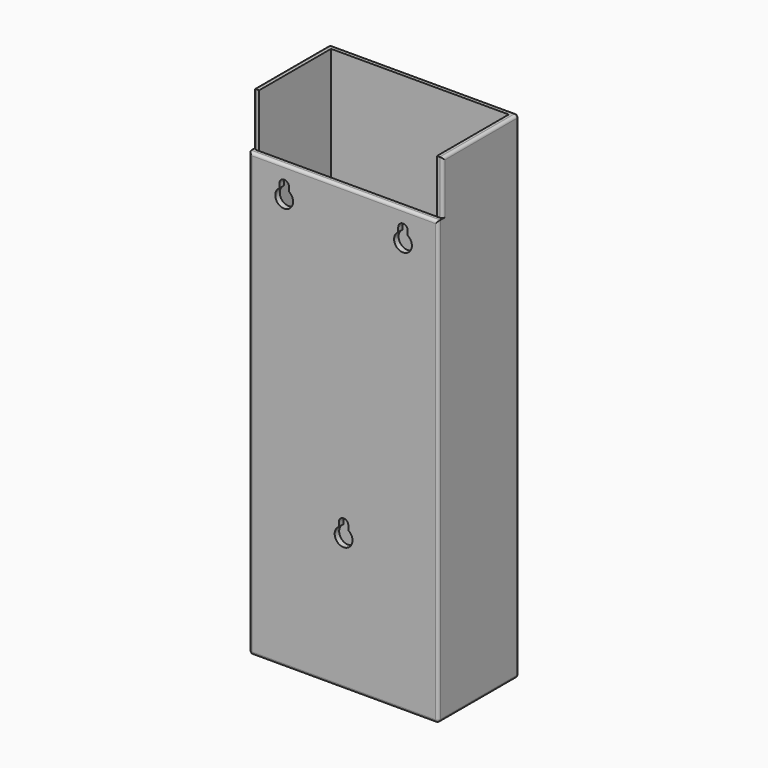
from build123d import *

# Parameters (mm, degrees)
F0_W     = 101
F0_H     = 54
F1_DEPTH = 132.5
F2_T     = -3
F3_W     = 101
F3_H     = 28.575
F4_DEPTH = 3
F6_DEPTH = 3
F7_R     = 1.5


with BuildPart() as f1:
    # F0 (on Top) → F1 (new body, symmetric)
    with BuildSketch(Plane.XY):
        Rectangle(F0_W, F0_H)
    extrude(amount=F1_DEPTH, both=True)

    # F2
    f2_openings = [f1.faces().sort_by_distance(p)[0] for p in [
        (0, 0, 132.5),
    ]]
    offset(amount=F2_T, openings=f2_openings)

    # F3 (on face) → F4 (cut, through all)
    with BuildSketch(Plane.XZ.offset(27)):
        with Locations((0, 118.2125)):
            Rectangle(F3_W, F3_H)
    extrude(amount=-F4_DEPTH, mode=Mode.SUBTRACT)

    # F5 (on face) → F6 (cut, through all)
    with BuildSketch(Plane.XZ.offset(27)):
        with BuildLine():
            Line((-34.29, 94.275), (-34.29, 91.9536233691))
            ThreePointArc((-34.29, 91.9536233691), (-31.75, 83.1625), (-29.21, 91.9536233691))
            Line((-29.21, 91.9536233691), (-29.21, 94.275))
            ThreePointArc((-29.21, 94.275), (-31.75, 96.815), (-34.29, 94.275))
        make_face()
        with BuildLine():
            ThreePointArc((34.29, 94.275), (31.75, 96.815), (29.21, 94.275))
            Line((29.21, 94.275), (29.21, 91.9536233691))
            ThreePointArc((29.21, 91.9536233691), (31.75, 83.1625), (34.29, 91.9536233691))
            Line((34.29, 91.9536233691), (34.29, 94.275))
        make_face()
        with BuildLine():
            Line((-2.54, -54.725), (-2.54, -57.0463766309))
            ThreePointArc((-2.54, -57.0463766309), (0, -65.8375), (2.54, -57.0463766309))
            Line((2.54, -57.0463766309), (2.54, -54.725))
            ThreePointArc((2.54, -54.725), (0, -52.185), (-2.54, -54.725))
        make_face()
    extrude(amount=-F6_DEPTH, mode=Mode.SUBTRACT)

    # F7
    f7_edges = [f1.edges().sort_by_distance(p)[0] for p in [
        (50.5, -27, -14.2875),
        (50.5, 27, 0),
        (-50.5, -27, -14.2875),
        (-50.5, 27, 0),
        (-50.5, 0, -132.5),
        (0, 27, -132.5),
        (0, -27, -132.5),
        (50.5, 0, -132.5),
        (-50.5, 1.5, 132.5),
        (0, 27, 132.5),
        (50.5, 1.5, 132.5),
        (0, -27, 103.925),
        (-50.5, -24, 118.2125),
        (50.5, -24, 118.2125),
    ]]
    fillet(f7_edges, radius=F7_R)


solid = f1.part
